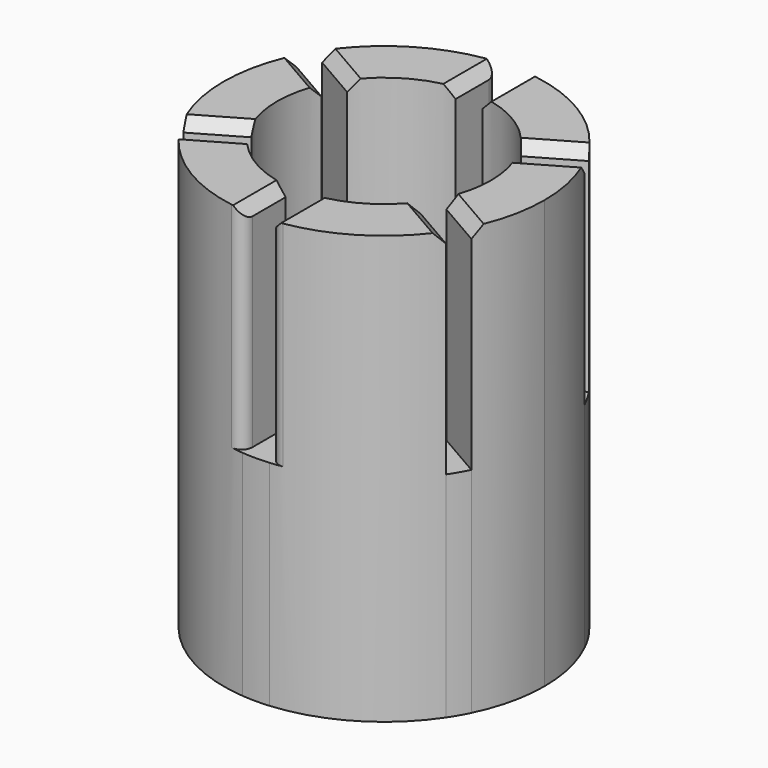
from build123d import *

# Parameters (mm, degrees)
F1_DEPTH    = 80
F0_R        = 10
F2_DEPTH    = 40
F0_R_2      = 4
F3_DEPTH    = 5
F4_SIZE     = 2
F5_T1_DEPTH = 43.847334297


# Not quite as in the source:
# - a fillet or chamfer that OpenCascade refuses, or shapes differently, is made with other operations: its cross-section is extruded or revolved along the edge and cut away or added


with BuildPart() as f1:
    # F0 (on Top) → F1 (new body)
    with BuildSketch(Plane.XY):
        with BuildLine():
            ThreePointArc((26.9229627936, -13.2345787395), (29.220616727, -6.7937881992), (30, 0))
            ThreePointArc((30, 0), (29.220616727, 6.7937881992), (26.9229627936, 13.2345787395))
            Line((26.9229627936, 13.2345787395), (18.2336879396, 8.2178235635))
            ThreePointArc((18.2336879396, 8.2178235635), (19.5534365112, 4.2027515515), (20, 0))
            ThreePointArc((20, 0), (19.5534365112, -4.2027515515), (18.2336879396, -8.2178235635))
            Line((18.2336879396, -8.2178235635), (26.9229627936, -13.2345787395))
        make_face()
    extrude(amount=F1_DEPTH)



with BuildPart() as f1b:
    # F0 (on Top) → F1, piece 2 (new body)
    with BuildSketch(Plane.XY):
        with BuildLine():
            Line((16.2336879396, 11.6819251786), (24.9229627936, 16.6986803547))
            ThreePointArc((24.9229627936, 16.6986803547), (15.21659411, 25.8545018071), (2.5, 29.8956518578))
            Line((2.5, 29.8956518578), (2.5, 19.843134833))
            ThreePointArc((2.5, 19.843134833), (10.2170984976, 17.1933387767), (16.2336879396, 11.6819251786))
        make_face()
    extrude(amount=F1_DEPTH)


with BuildPart() as f1c:
    # F0 (on Top) → F1, piece 3 (new body)
    with BuildSketch(Plane.XY):
        with BuildLine():
            ThreePointArc((2.5, -29.8956518578), (15.21659411, -25.8545018071), (24.9229627936, -16.6986803547))
            Line((24.9229627936, -16.6986803547), (16.2336879396, -11.6819251786))
            ThreePointArc((16.2336879396, -11.6819251786), (10.2170984976, -17.1933387767), (2.5, -19.843134833))
            Line((2.5, -19.843134833), (2.5, -29.8956518578))
        make_face()
    extrude(amount=F1_DEPTH)


with BuildPart() as f1d:
    # F0 (on Top) → F1, piece 4 (new body)
    with BuildSketch(Plane.XY):
        with BuildLine():
            Line((-2.5, 19.843134833), (-2.5, 29.8956518578))
            ThreePointArc((-2.5, 29.8956518578), (-15.21659411, 25.8545018071), (-24.9229627936, 16.6986803547))
            Line((-24.9229627936, 16.6986803547), (-16.2336879396, 11.6819251786))
            ThreePointArc((-16.2336879396, 11.6819251786), (-10.2170984976, 17.1933387767), (-2.5, 19.843134833))
        make_face()
    extrude(amount=F1_DEPTH)


with BuildPart() as f1e:
    # F0 (on Top) → F1, piece 5 (new body)
    with BuildSketch(Plane.XY):
        with BuildLine():
            ThreePointArc((-24.9229627936, -16.6986803547), (-15.21659411, -25.8545018071), (-2.5, -29.8956518578))
            Line((-2.5, -29.8956518578), (-2.5, -19.843134833))
            ThreePointArc((-2.5, -19.843134833), (-10.2170984976, -17.1933387767), (-16.2336879396, -11.6819251786))
            Line((-16.2336879396, -11.6819251786), (-24.9229627936, -16.6986803547))
        make_face()
    extrude(amount=F1_DEPTH)


with BuildPart() as f1f:
    # F0 (on Top) → F1, piece 6 (new body)
    with BuildSketch(Plane.XY):
        with BuildLine():
            Line((-18.2336879396, 8.2178235635), (-26.9229627936, 13.2345787395))
            ThreePointArc((-26.9229627936, 13.2345787395), (-30, 0), (-26.9229627936, -13.2345787395))
            Line((-26.9229627936, -13.2345787395), (-18.2336879396, -8.2178235635))
            ThreePointArc((-18.2336879396, -8.2178235635), (-20, 0), (-18.2336879396, 8.2178235635))
        make_face()
    extrude(amount=F1_DEPTH)


with BuildPart() as f1_1:
    add(f1.part)

    add(f1b.part)  # F2 merges F1b

    add(f1c.part)  # F2 merges F1c

    add(f1d.part)  # F2 merges F1d

    add(f1e.part)  # F2 merges F1e

    add(f1f.part)  # F2 merges F1f
    # F0 (on Top) → F2 (join)
    with BuildSketch(Plane.XY):
        with BuildLine():
            Line((18.2336879396, 8.2178235635), (26.9229627936, 13.2345787395))
            ThreePointArc((26.9229627936, 13.2345787395), (25.9807621135, 15), (24.9229627936, 16.6986803547))
            Line((24.9229627936, 16.6986803547), (16.2336879396, 11.6819251786))
            ThreePointArc((16.2336879396, 11.6819251786), (17.3205080757, 10), (18.2336879396, 8.2178235635))
        make_face()
        with BuildLine():
            ThreePointArc((24.9229627936, -16.6986803547), (25.9807621135, -15), (26.9229627936, -13.2345787395))
            Line((26.9229627936, -13.2345787395), (18.2336879396, -8.2178235635))
            ThreePointArc((18.2336879396, -8.2178235635), (17.3205080757, -10), (16.2336879396, -11.6819251786))
            Line((16.2336879396, -11.6819251786), (24.9229627936, -16.6986803547))
        make_face()
        with BuildLine():
            ThreePointArc((20, 0), (19.5534365112, 4.2027515515), (18.2336879396, 8.2178235635))
            ThreePointArc((18.2336879396, 8.2178235635), (17.3205080757, 10), (16.2336879396, 11.6819251786))
            ThreePointArc((16.2336879396, 11.6819251786), (10.2170984976, 17.1933387767), (2.5, 19.843134833))
            ThreePointArc((2.5, 19.843134833), (0, 20), (-2.5, 19.843134833))
            ThreePointArc((-2.5, 19.843134833), (-10.2170984976, 17.1933387767), (-16.2336879396, 11.6819251786))
            ThreePointArc((-16.2336879396, 11.6819251786), (-17.3205080757, 10), (-18.2336879396, 8.2178235635))
            ThreePointArc((-18.2336879396, 8.2178235635), (-20, 0), (-18.2336879396, -8.2178235635))
            ThreePointArc((-18.2336879396, -8.2178235635), (-17.3205080757, -10), (-16.2336879396, -11.6819251786))
            ThreePointArc((-16.2336879396, -11.6819251786), (-10.2170984976, -17.1933387767), (-2.5, -19.843134833))
            ThreePointArc((-2.5, -19.843134833), (0, -20), (2.5, -19.843134833))
            ThreePointArc((2.5, -19.843134833), (10.2170984976, -17.1933387767), (16.2336879396, -11.6819251786))
            ThreePointArc((16.2336879396, -11.6819251786), (17.3205080757, -10), (18.2336879396, -8.2178235635))
            ThreePointArc((18.2336879396, -8.2178235635), (19.5534365112, -4.2027515515), (20, 0))
        make_face()
        Circle(F0_R, mode=Mode.SUBTRACT)
        with BuildLine():
            Line((2.5, 19.843134833), (2.5, 29.8956518578))
            ThreePointArc((2.5, 29.8956518578), (0, 30), (-2.5, 29.8956518578))
            Line((-2.5, 29.8956518578), (-2.5, 19.843134833))
            ThreePointArc((-2.5, 19.843134833), (0, 20), (2.5, 19.843134833))
        make_face()
        with BuildLine():
            ThreePointArc((-2.5, -29.8956518578), (0, -30), (2.5, -29.8956518578))
            Line((2.5, -29.8956518578), (2.5, -19.843134833))
            ThreePointArc((2.5, -19.843134833), (0, -20), (-2.5, -19.843134833))
            Line((-2.5, -19.843134833), (-2.5, -29.8956518578))
        make_face()
        with BuildLine():
            Line((-16.2336879396, 11.6819251786), (-24.9229627936, 16.6986803547))
            ThreePointArc((-24.9229627936, 16.6986803547), (-25.9807621135, 15), (-26.9229627936, 13.2345787395))
            Line((-26.9229627936, 13.2345787395), (-18.2336879396, 8.2178235635))
            ThreePointArc((-18.2336879396, 8.2178235635), (-17.3205080757, 10), (-16.2336879396, 11.6819251786))
        make_face()
        with BuildLine():
            ThreePointArc((-26.9229627936, -13.2345787395), (-25.9807621135, -15), (-24.9229627936, -16.6986803547))
            Line((-24.9229627936, -16.6986803547), (-16.2336879396, -11.6819251786))
            ThreePointArc((-16.2336879396, -11.6819251786), (-17.3205080757, -10), (-18.2336879396, -8.2178235635))
            Line((-18.2336879396, -8.2178235635), (-26.9229627936, -13.2345787395))
        make_face()
    extrude(amount=F2_DEPTH)

    # F0 (on Top) → F3 (join)
    with BuildSketch(Plane.XY):
        Circle(F0_R)
        Circle(F0_R_2, mode=Mode.SUBTRACT)
    extrude(amount=F3_DEPTH)

    # F4
    f4_edges = [f1_1.edges().sort_by_distance(p)[0] for p in [
        (-20.578325, 14.190303, 80),
        (-22.578325, 10.726201, 80),
        (-22.578325, -10.726201, 80),
        (-20.578325, -14.190303, 80),
        (20.578325, -14.190303, 80),
        (22.578325, -10.726201, 80),
        (22.578325, 10.726201, 80),
        (20.578325, 14.190303, 80),
        (-2.5, 24.869393, 80),
        (2.5, 24.869393, 80),
        (2.5, -24.869393, 80),
        (-2.5, -24.869393, 80),
    ]]
    chamfer(f4_edges, length=F4_SIZE)

    # F5: fillet of radius 2 on 6 edges, made by hand

    # F5_s2 → F5_t1 (cut)
    with BuildSketch(Plane.XY.offset(40)):
        with BuildLine():
            ThreePointArc((-2.5, 27.6360272109), (-3.2044030609, 29.1596507114), (-4.8214285714, 29.6100291545))
            ThreePointArc((-4.8214285714, 29.6100291545), (-3.6634988964, 29.7754727223), (-2.5, 29.8956518578))
            Line((-2.5, 29.8956518578), (-2.5, 27.6360272109))
        make_face()
        with BuildLine():
            ThreePointArc((4.8214285714, 29.6100291545), (3.2044030609, 29.1596507114), (2.5, 27.6360272109))
            Line((2.5, 27.6360272109), (2.5, 29.8956518578))
            ThreePointArc((2.5, 29.8956518578), (3.6634988964, 29.7754727223), (4.8214285714, 29.6100291545))
        make_face()
        with BuildLine():
            ThreePointArc((-4.8214285714, -29.6100291545), (-3.2044030609, -29.1596507114), (-2.5, -27.6360272109))
            Line((-2.5, -27.6360272109), (-2.5, -29.8956518578))
            ThreePointArc((-2.5, -29.8956518578), (-3.6634988964, -29.7754727223), (-4.8214285714, -29.6100291545))
        make_face()
        with BuildLine():
            ThreePointArc((4.8214285714, -29.6100291545), (3.2044030609, -29.1596507114), (2.5, -27.6360272109))
            Line((2.5, -27.6360272109), (2.5, -29.8956518578))
            ThreePointArc((2.5, -29.8956518578), (3.6634988964, -29.7754727223), (4.8214285714, -29.6100291545))
        make_face()
    extrude(amount=F5_T1_DEPTH, mode=Mode.SUBTRACT)


solid = f1_1.part
